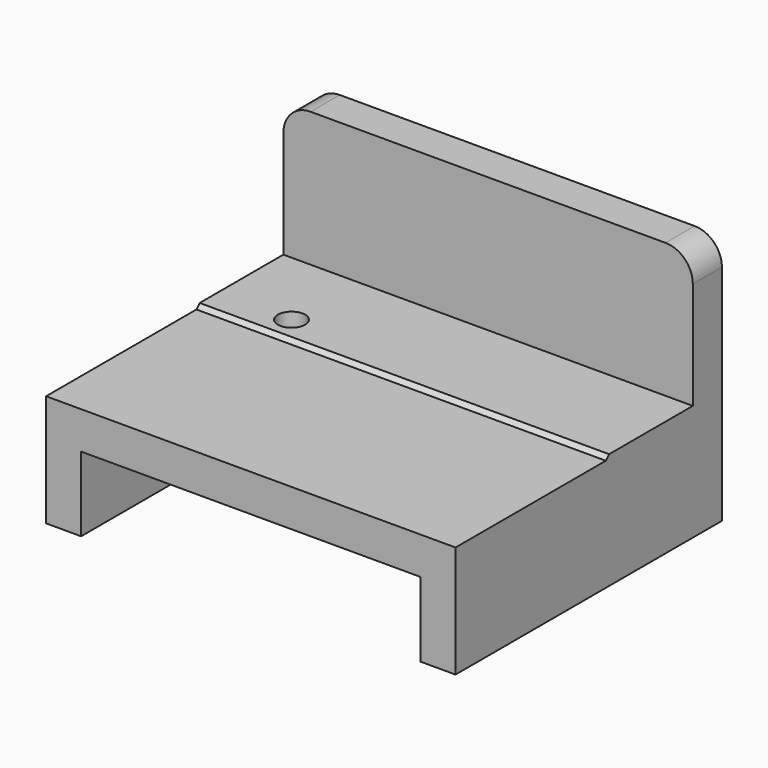
from build123d import *

# Parameters (mm, degrees)
F0_W        = 45
F0_H        = 36.6
F1_DEPTH    = 12.3
F2_W        = 37.3
F2_H        = 8.2
F3_DEPTH    = 36.601
F4_W        = 45
F4_H        = 16
F5_DEPTH    = 0.45
F6_T4_DEPTH = 47.571682988
F7_W        = 45
F7_H        = 4
F8_DEPTH    = 14.8
F9_R        = 3
F10_W       = 8.5
F10_H       = 4
F11_DEPTH   = 10.8
F12_R       = 3
F13_R       = 1.5
F14_DEPTH   = 25
F15_R       = 1.5
F16_DEPTH   = 25


# Not quite as in the source:
# - a fillet or chamfer that OpenCascade refuses, or shapes differently, is made with other operations: its cross-section is extruded or revolved along the edge and cut away or added


with BuildPart() as f1:
    # F0 (on Top) → F1 (new body)
    with BuildSketch(Plane.XY):
        Rectangle(F0_W, F0_H)
    extrude(amount=F1_DEPTH)

    # F2 (on face) → F3 (cut, through all)
    with BuildSketch(Plane.XZ.offset(18.3)):
        with Locations((0, 4.1)):
            Rectangle(F2_W, F2_H)
    extrude(amount=-F3_DEPTH, mode=Mode.SUBTRACT)

    # F4 (on face) → F5 (join)
    with BuildSketch(Plane.XY.offset(12.3)):
        with Locations((0, 10.3)):
            Rectangle(F4_W, F4_H)
    extrude(amount=F5_DEPTH)

    # F6: chamfer of 0.5 on 1 edges, made by hand


with BuildPart() as f6_tool2:
    # F6_s3 → F6_t4 (new body)
    with BuildSketch(Plane.YZ.offset(-23.785841494)):
        Polygon((2.3, 12.25), (2.8, 12.75), (2.3, 12.75), align=None)
    extrude(amount=F6_T4_DEPTH)

    split(bisect_by=Plane.XY.offset(12.3), keep=Keep.TOP)


with BuildPart() as f1_1:
    add(f1.part)

    # F6_t1: cut F6_tool2
    add(f6_tool2.part, mode=Mode.SUBTRACT)

    # F7 (on face) → F8 (join)
    with BuildSketch(Plane.XY.offset(12.75)):
        with Locations((0, 16.3)):
            Rectangle(F7_W, F7_H)
    extrude(amount=F8_DEPTH)

    # F9
    f9_edges = [f1_1.edges().sort_by_distance(p)[0] for p in [
        (-22.5, 16.3, 27.55),
        (22.5, 16.3, 27.55),
    ]]
    fillet(f9_edges, radius=F9_R)

    # F10 (on face) → F11 (join)
    with BuildSketch(Plane(origin=(0, 18.3, 0), x_dir=(-1, 0, 0), z_dir=(0, 1, 0))):
        with Locations((14.4, 10.2)):
            Rectangle(F10_W, F10_H)
    extrude(amount=F11_DEPTH)

    # F12
    f12_edges = [f1_1.edges().sort_by_distance(p)[0] for p in [
        (-10.15, 29.1, 10.2),
        (-18.65, 29.1, 10.2),
    ]]
    fillet(f12_edges, radius=F12_R)

    # F13 (on face) → F14 (cut)
    with BuildSketch(Plane.XY.offset(12.2)):
        with Locations((-14.4, 25.3)):
            Circle(F13_R)
        with Locations((-14.4, 20.3)):
            Circle(F13_R)
    extrude(amount=-F14_DEPTH, mode=Mode.SUBTRACT)

    # F15 (on face) → F16 (cut)
    with BuildSketch(Plane.XY.offset(12.75)):
        with Locations((-14.4, 5.2980469912)):
            Circle(F15_R)
    extrude(amount=-F16_DEPTH, mode=Mode.SUBTRACT)


solid = f1_1.part
